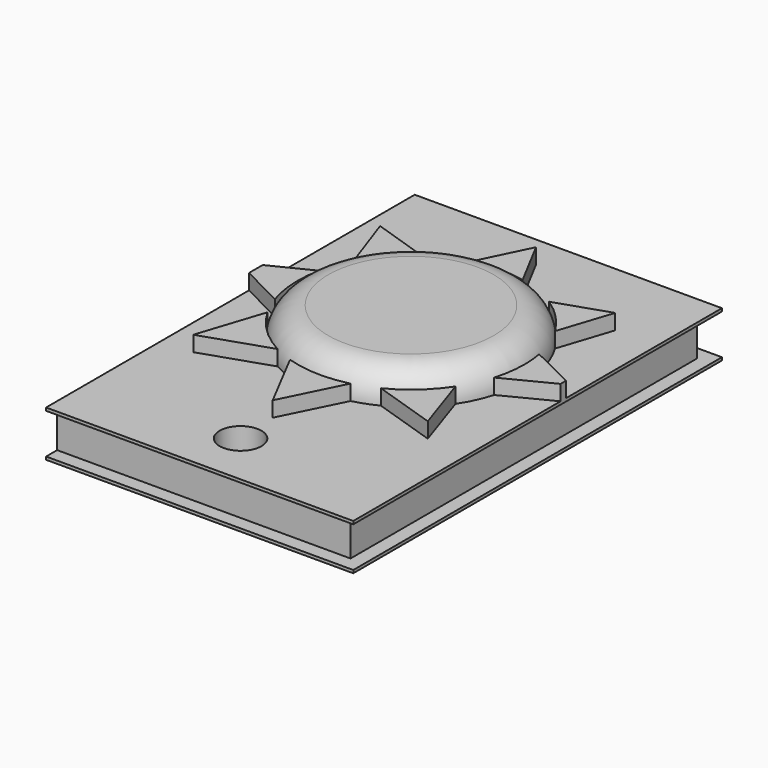
from build123d import *

# Parameters (mm, degrees)
F0_W      = 50.8
F0_H      = 76.2
F1_DEPTH  = 7.62
F2_R      = 18.7529717457
F3_DEPTH  = 5.08
F4_R      = 5.07999
F7_DEPTH  = 2.54
F8_W      = 50.2787431046
F8_H      = 6.6451809329
F9_DEPTH  = 2.286
F10_W     = 73.914
F10_H     = 6.6451809329
F11_DEPTH = 2.286
F12_W     = 48.514
F12_H     = 6.6451809329
F13_DEPTH = 2.286
F14_R     = 3.4596539052
F15_DEPTH = 25.4


# Not quite as in the source:
# - a fillet or chamfer is up to 0.001 mm smaller than in the source, because OpenCascade refuses the exact size


with BuildPart() as f1:
    # F0 (on Top) → F1 (new body)
    with BuildSketch(Plane.XY):
        with Locations((0.3819083795, -6.0587156958)):
            Rectangle(F0_W, F0_H)
    extrude(amount=F1_DEPTH)

    # F2 (on face) → F3 (join)
    with BuildSketch(Plane.XY.offset(7.62)):
        Circle(F2_R)
    extrude(amount=F3_DEPTH)

    # F4 (radius 5.08 in the source; OpenCascade refuses exactly that, so slightly less here)
    f4_edges = [f1.edges().sort_by_distance(p)[0] for p in [
        (-18.752972, 0, 12.7),
    ]]
    fillet(f4_edges, radius=F4_R)

    # F5 (on face) + F6 (on face) → F7 (join)
    with BuildSketch(Plane.XY.offset(7.62)):
        with BuildLine():
            ThreePointArc((-17.8012941845, -5.8981246722), (-18.7253311698, -1.0178024727), (-18.33570835, 3.9339228004))
            Line((-18.33570835, 3.9339228004), (-25.0180916205, 0.604446249))
            Line((-25.0180916205, 0.604446249), (-25.0180916205, -2.1975415816))
            Line((-25.0180916205, -2.1975415816), (-17.8012941845, -5.8981246722))
        make_face()
        with BuildLine():
            Line((-0.56613778, 26.5454184264), (-4.6479069665, 18.1678537567))
            ThreePointArc((-4.6479069665, 18.1678537567), (-0.450512239, 18.7475595216), (3.7698827091, 18.3701370069))
            Line((3.7698827091, 18.3701370069), (-0.56613778, 26.5454184264))
        make_face()
        with BuildLine():
            Line((18.8934579492, 18.5859743506), (10.2606709283, 15.6968971901))
            ThreePointArc((10.2606709283, 15.6968971901), (13.4651875999, 13.0523052444), (16.0087319261, 9.7670083143))
            Line((16.0087319261, 9.7670083143), (18.8934579492, 18.5859743506))
        make_face()
        with BuildLine():
            Line((25.7819083795, -1.3151803242), (25.7819083795, -0.2086242448))
            Line((25.7819083795, -0.2086242448), (18.4334550561, 3.4469818664))
            ThreePointArc((18.4334550561, 3.4469818664), (18.6729217202, 1.7308794659), (18.7529717457, 0))
            ThreePointArc((18.7529717457, 0), (18.5619015059, -2.6701613771), (17.9925843387, -5.2859112847))
            Line((17.9925843387, -5.2859112847), (25.7819083795, -1.3151803242))
        make_face()
        with BuildLine():
            ThreePointArc((15.6345242212, -10.3554624074), (12.4475757879, -14.0261115887), (8.4242275529, -16.7542931642))
            Line((8.4242275529, -16.7542931642), (18.9255586046, -20.1893288404))
            Line((18.9255586046, -20.1893288404), (15.6345242212, -10.3554624074))
        make_face()
        with BuildLine():
            ThreePointArc((4.5489366376, -18.1928866528), (-0.6058031571, -18.7431841433), (-5.7142487726, -17.8611676623))
            Line((-5.7142487726, -17.8611676623), (-0.3793946235, -28.119046241))
            Line((-0.3793946235, -28.119046241), (4.5489366376, -18.1928866528))
        make_face()
        with BuildLine():
            ThreePointArc((-8.8478629176, -16.5344873245), (-13.0678043341, -13.4501464371), (-16.2725260484, -9.3208822167))
            Line((-16.2725260484, -9.3208822167), (-19.8348792175, -20.2114386703))
            Line((-19.8348792175, -20.2114386703), (-8.8478629176, -16.5344873245))
        make_face()
    with BuildSketch(Plane.XY.offset(7.62)):
        with BuildLine():
            Line((-10.5754289904, 15.4865829337), (-19.9908912182, 18.6000298709))
            Line((-19.9908912182, 18.6000298709), (-16.5623554019, 8.7955859859))
            ThreePointArc((-16.5623554019, 8.7955859859), (-13.9752350774, 12.5046692809), (-10.5754289904, 15.4865829337))
        make_face()
    extrude(amount=F7_DEPTH)

    # F8 (on face) → F9 (cut)
    with BuildSketch(Plane(origin=(0, 32.0412843042, 0), x_dir=(-1, 0, 0), z_dir=(0, 1, 0))):
        with Locations((-0.6425368272, 3.8051904665)):
            Rectangle(F8_W, F8_H)
    extrude(amount=-F9_DEPTH, mode=Mode.SUBTRACT)

    # F10 (on face) → F11 (cut)
    with BuildSketch(Plane.YZ.offset(25.7819083795)):
        with Locations((-7.2017156958, 3.8051904665)):
            Rectangle(F10_W, F10_H)
    extrude(amount=-F11_DEPTH, mode=Mode.SUBTRACT)

    # F12 (on face) → F13 (cut)
    with BuildSketch(Plane.XZ.offset(44.1587156958)):
        with Locations((-0.7610916205, 3.8051904665)):
            Rectangle(F12_W, F12_H)
    extrude(amount=-F13_DEPTH, mode=Mode.SUBTRACT)

    # F14 (on face) → F15 (cut)
    with BuildSketch(Plane.XY.offset(7.62)):
        with Locations((0, -35.2311357856)):
            Circle(F14_R)
    extrude(amount=-F15_DEPTH, mode=Mode.SUBTRACT)


solid = f1.part
